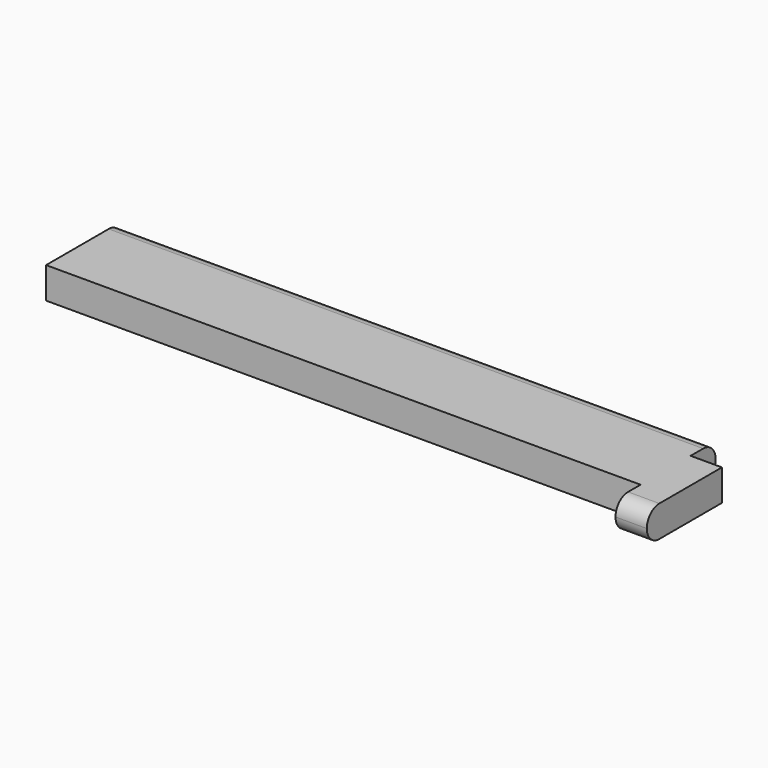
from build123d import *

# Parameters (mm, degrees)
F1_DEPTH = 2.5
F2_R     = 2.49999


# Not quite as in the source:
# - a fillet or chamfer is up to 0.001 mm smaller than in the source, because OpenCascade refuses the exact size


with BuildPart() as f1:
    # F0 (on Top) → F1 (new body, symmetric)
    with BuildSketch(Plane.XY):
        Polygon((95, 7.5), (0, 7.5), (0, -7.5), (95, -7.5), (95, -12.5), (100, -12.5), (100, 2.5), (95, 2.5), align=None)
    extrude(amount=F1_DEPTH, both=True)

    # F2 (radius 2.5 in the source; OpenCascade refuses exactly that, so slightly less here)
    f2_edges = [f1.edges().sort_by_distance(p)[0] for p in [
        (97.5, -12.5, 2.5),
        (97.5, -12.5, -2.5),
        (47.5, 7.5, 2.5),
        (47.5, 7.5, -2.5),
    ]]
    fillet(f2_edges, radius=F2_R)


solid = f1.part
